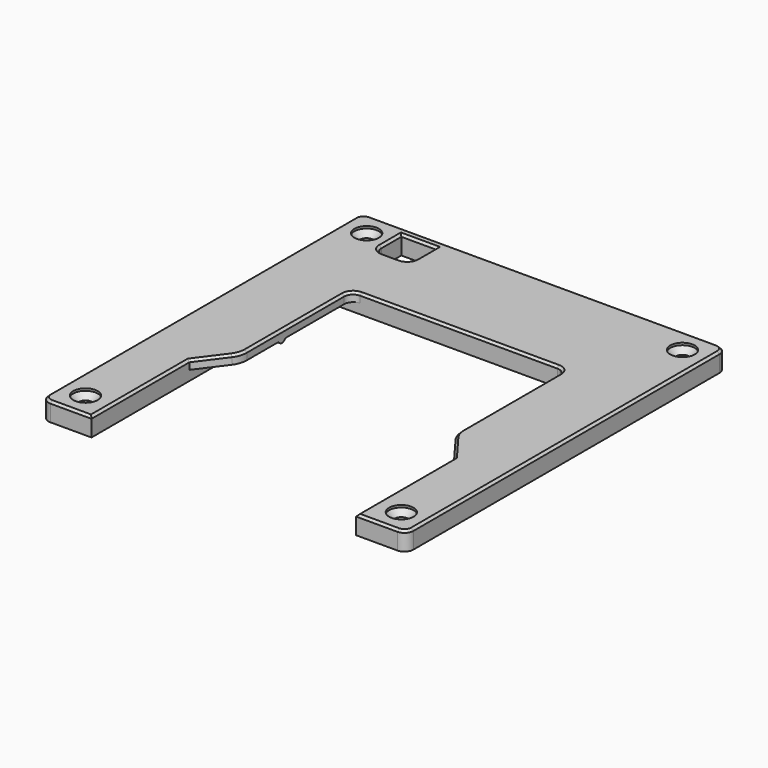
from build123d import *

# Parameters (mm, degrees)
F1_DEPTH      = 2
F3_DEPTH      = 2.2
F5_DEPTH      = 25
F6_R          = 1.5
F7_DEPTH      = 4.2
F8_R          = 2.75
F9_DEPTH      = 2
F10_S5_R      = 1.5
F10_T6_DEPTH  = 5
F10_S11_R     = 1.5
F10_T12_DEPTH = 5
F10_S17_R     = 1.5
F10_T18_DEPTH = 5
F10_S23_R     = 1.5
F10_T24_DEPTH = 5
F11_W         = 5.6
F11_H         = 2
F12_DEPTH     = 0.6
F13_T1_DEPTH  = 8.4722813233
F13_T3_DEPTH  = 8.4722813233
F14_SIZE      = 0.5


# Not quite as in the source:
# - a fillet or chamfer that OpenCascade refuses, or shapes differently, is made with other operations: its cross-section is extruded or revolved along the edge and cut away or added


with BuildPart() as f1:
    # F0 (on Top) → F1 (new body)
    with BuildSketch(Plane.XY):
        with BuildLine():
            Line((80, 0), (2, 0))
            ThreePointArc((2, 0), (0.5857864376, -0.5857864376), (0, -2))
            Line((0, -2), (0, -88))
            ThreePointArc((0, -88), (0.5857864376, -89.4142135624), (2, -90))
            Line((2, -90), (11.25, -90))
            Line((11.25, -90), (11.25, -62.5))
            Line((11.25, -62.5), (15.8564011104, -56.3307127986))
            ThreePointArc((15.8564011104, -56.3307127986), (16.5951030311, -54.9153368199), (16.85, -53.3392666362))
            Line((16.85, -53.3392666362), (16.85, -26))
            ThreePointArc((16.85, -26), (17.4357864376, -24.5857864376), (18.85, -24))
            Line((18.85, -24), (63.15, -24))
            ThreePointArc((63.15, -24), (64.5642135624, -24.5857864376), (65.15, -26))
            Line((65.15, -26), (65.15, -53.3392666362))
            ThreePointArc((65.15, -53.3392666362), (65.4048969689, -54.9153368199), (66.1435988896, -56.3307127986))
            Line((66.1435988896, -56.3307127986), (70.75, -62.5))
            Line((70.75, -62.5), (70.75, -90))
            Line((70.75, -90), (80, -90))
            ThreePointArc((80, -90), (81.4142135624, -89.4142135624), (82, -88))
            Line((82, -88), (82, -2))
            ThreePointArc((82, -2), (81.4142135624, -0.5857864376), (80, 0))
        make_face()
    extrude(amount=F1_DEPTH)

    # F2 (on face) → F3 (join)
    with BuildSketch(Plane(origin=(0, 0, 0), x_dir=(1, 0, 0), z_dir=(0, 0, -1))):
        with BuildLine():
            ThreePointArc((80, 0), (81.4142135624, 0.5857864376), (82, 2))
            Line((82, 2), (82, 88))
            ThreePointArc((82, 88), (81.4142135624, 89.4142135624), (80, 90))
            Line((80, 90), (70.75, 90))
            Line((70.75, 90), (70.75, 62.5))
            Line((70.75, 62.5), (70.75, 26))
            ThreePointArc((70.75, 26), (70.1642135624, 24.5857864376), (68.75, 24))
            Line((68.75, 24), (65.15, 24))
            Line((65.15, 24), (16.85, 24))
            Line((16.85, 24), (13.25, 24))
            ThreePointArc((13.25, 24), (11.8357864376, 24.5857864376), (11.25, 26))
            Line((11.25, 26), (11.25, 62.5))
            Line((11.25, 62.5), (11.25, 90))
            Line((11.25, 90), (2, 90))
            ThreePointArc((2, 90), (0.5857864376, 89.4142135624), (0, 88))
            Line((0, 88), (0, 2))
            ThreePointArc((0, 2), (0.5857864376, 0.5857864376), (2, 0))
            Line((2, 0), (80, 0))
        make_face()
    extrude(amount=F3_DEPTH)

    # F4 (on face) → F5 (cut)
    with BuildSketch(Plane.XY.offset(2)):
        with BuildLine():
            Line((18.3, -2), (10.5, -2))
            Line((10.5, -2), (10.5, -7.6))
            ThreePointArc((10.5, -7.6), (11.0857864376, -9.0142135624), (12.5, -9.6))
            Line((12.5, -9.6), (16.3, -9.6))
            ThreePointArc((16.3, -9.6), (17.7142135624, -9.0142135624), (18.3, -7.6))
            Line((18.3, -7.6), (18.3, -2))
        make_face()
    extrude(amount=-F5_DEPTH, mode=Mode.SUBTRACT)

    # F6 (on face) → F7 (cut)
    with BuildSketch(Plane.XY.offset(2)):
        with Locations((5.5, -84.5)):
            Circle(F6_R)
        with Locations((76.5, -84.5)):
            Circle(F6_R)
        with Locations((5.5, -5.5)):
            Circle(F6_R)
        with Locations((76.5, -5.5)):
            Circle(F6_R)
    extrude(amount=-F7_DEPTH, mode=Mode.SUBTRACT)

    # F8 (on face) → F9 (cut)
    with BuildSketch(Plane.XY.offset(2)):
        with Locations((5.5, -5.5)):
            Circle(F8_R)
        with Locations((76.5, -5.5)):
            Circle(F8_R)
        with Locations((76.5, -84.5)):
            Circle(F8_R)
        with Locations((5.5, -84.5)):
            Circle(F8_R)
    extrude(amount=-F9_DEPTH, mode=Mode.SUBTRACT)

    # F10: chamfer of 1.5 on 4 edges, made by hand


with BuildPart() as f10_tool2:
    # F10_s3 → F10_t4 (revolve)
    with BuildSketch(Plane.XZ.offset(84.5)):
        Polygon((8.25, 1.5), (6.75, 0), (8.25, 0), align=None)
    revolve(axis=Axis((5.5, -84.5, 0), (0, 0, 1)))

    # F10_s5 → F10_t6 (cut, symmetric)
    with BuildSketch(Plane.XY.offset(0.7)):
        with Locations((5.5, -84.5)):
            Circle(F10_S5_R)
    extrude(amount=F10_T6_DEPTH, both=True, mode=Mode.SUBTRACT)


with BuildPart() as f1_1:
    add(f1.part)

    # F10_t1: union F10_tool2
    add(f10_tool2.part)


with BuildPart() as f10_tool8:
    # F10_s9 → F10_t10 (revolve)
    with BuildSketch(Plane.XZ.offset(84.5)):
        Polygon((79.25, 1.5), (77.75, 0), (79.25, 0), align=None)
    revolve(axis=Axis((76.5, -84.5, 0), (0, 0, 1)))

    # F10_s11 → F10_t12 (cut, symmetric)
    with BuildSketch(Plane.XY.offset(0.7)):
        with Locations((76.5, -84.5)):
            Circle(F10_S11_R)
    extrude(amount=F10_T12_DEPTH, both=True, mode=Mode.SUBTRACT)


with BuildPart() as f1_2:
    add(f1_1.part)

    # F10_t7: union F10_tool8
    add(f10_tool8.part)


with BuildPart() as f10_tool14:
    # F10_s15 → F10_t16 (revolve)
    with BuildSketch(Plane.XZ.offset(5.5)):
        Polygon((8.25, 1.5), (6.75, 0), (8.25, 0), align=None)
    revolve(axis=Axis((5.5, -5.5, 0), (0, 0, 1)))

    # F10_s17 → F10_t18 (cut, symmetric)
    with BuildSketch(Plane.XY.offset(0.7)):
        with Locations((5.5, -5.5)):
            Circle(F10_S17_R)
    extrude(amount=F10_T18_DEPTH, both=True, mode=Mode.SUBTRACT)


with BuildPart() as f1_3:
    add(f1_2.part)

    # F10_t13: union F10_tool14
    add(f10_tool14.part)


with BuildPart() as f10_tool20:
    # F10_s21 → F10_t22 (revolve)
    with BuildSketch(Plane.XZ.offset(5.5)):
        Polygon((79.25, 1.5), (77.75, 0), (79.25, 0), align=None)
    revolve(axis=Axis((76.5, -5.5, 0), (0, 0, 1)))

    # F10_s23 → F10_t24 (cut, symmetric)
    with BuildSketch(Plane.XY.offset(0.7)):
        with Locations((76.5, -5.5)):
            Circle(F10_S23_R)
    extrude(amount=F10_T24_DEPTH, both=True, mode=Mode.SUBTRACT)


with BuildPart() as f1_4:
    add(f1_3.part)

    # F10_t19: union F10_tool20
    add(f10_tool20.part)

    # F11 (on face) → F12 (join)
    with BuildSketch(Plane(origin=(0, 0, 0), x_dir=(1, 0, 0), z_dir=(0, 0, -1))):
        with Locations((14.05, 43.5)):
            Rectangle(F11_W, F11_H)
        with Locations((67.95, 43.5)):
            Rectangle(F11_W, F11_H)
    extrude(amount=F12_DEPTH)

    # F13: fillet of radius 1.4 on 4 edges, made by hand

    # F13_s2 → F13_t1 (cut)
    with BuildSketch(Plane.YZ.offset(11.25)):
        with BuildLine():
            ThreePointArc((-42.5, 0), (-43.0008384595, -0.4409673646), (-43.6489125293, -0.6))
            Line((-43.6489125293, -0.6), (-42.5, -0.6))
            Line((-42.5, -0.6), (-42.5, 0))
        make_face()
        with BuildLine():
            ThreePointArc((-43.3510874707, -0.6), (-43.9991615405, -0.4409673646), (-44.5, 0))
            Line((-44.5, 0), (-44.5, -0.6))
            Line((-44.5, -0.6), (-43.3510874707, -0.6))
        make_face()
    extrude(amount=F13_T1_DEPTH, mode=Mode.SUBTRACT)

    # F13_s4 → F13_t3 (cut)
    with BuildSketch(Plane.YZ.offset(62.2777186767)):
        with BuildLine():
            ThreePointArc((-43.6489125293, -0.6), (-43.0008384595, -0.4409673646), (-42.5, 0))
            Line((-42.5, 0), (-42.5, -0.6))
            Line((-42.5, -0.6), (-43.6489125293, -0.6))
        make_face()
        with BuildLine():
            ThreePointArc((-44.5, 0), (-43.9991615405, -0.4409673646), (-43.3510874707, -0.6))
            Line((-43.3510874707, -0.6), (-44.5, -0.6))
            Line((-44.5, -0.6), (-44.5, 0))
        make_face()
    extrude(amount=F13_T3_DEPTH, mode=Mode.SUBTRACT)

    # F14
    f14_edges = [f1_4.edges().sort_by_distance(p)[0] for p in [
        (0.585786, -0.585786, 2),
        (41, 0, 2),
        (0, -45, 2),
        (10.5, -4.8, 2),
        (14.4, -2, 2),
        (18.3, -4.8, 2),
        (17.714214, -9.014214, 2),
        (14.4, -9.6, 2),
        (11.085786, -9.014214, 2),
        (81.414214, -0.585786, 2),
        (82, -45, 2),
        (11.25, -76.25, 2),
        (6.625, -90, 2),
        (0.585786, -89.414214, 2),
        (81.414214, -89.414214, 2),
        (75.375, -90, 2),
        (70.75, -76.25, 2),
        (68.446799, -59.415356, 2),
        (65.404897, -54.915337, 2),
        (65.15, -39.669633, 2),
        (64.564214, -24.585786, 2),
        (41, -24, 2),
        (17.435786, -24.585786, 2),
        (16.85, -39.669633, 2),
        (16.595103, -54.915337, 2),
        (13.553201, -59.415356, 2),
    ]]
    chamfer(f14_edges, length=F14_SIZE)


solid = f1_4.part
